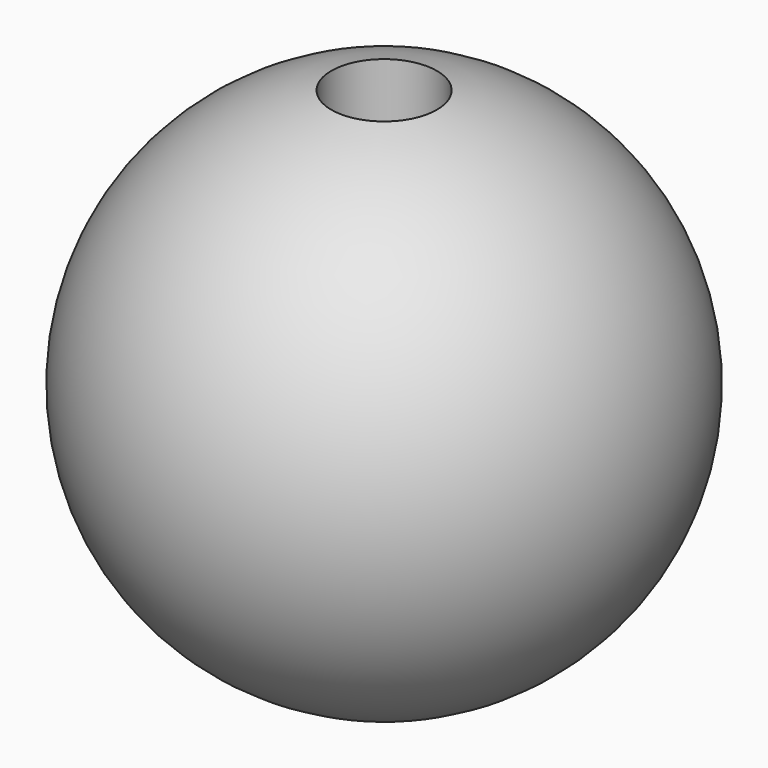
from build123d import *

# Parameters (mm, degrees)
F4_R         = 3.175
F5_DEPTH     = 50.8
F7_ANGLE     = 105.1
F9_TEXT_SIZE = 3.7345061881
F10_DEPTH    = 19.05


# Not quite as in the source:
# - Text() gives the source's letters only with a copy of the font that has no kerning and outlines rounded to 1/6400 em; it was checked with that copy


with BuildPart() as f2:
    # F0 (on Front) → F2 (revolve)
    with BuildSketch(Plane.XZ):
        with BuildLine():
            Line((0, -15.875), (0, 15.875))
            ThreePointArc((0, 15.875), (-15.875, 0), (0, -15.875))
        make_face()
    revolve(axis=Axis((0, 0, 0), (0, 0, 1)))

    # F9 (on offset) → F10 (cut)
    with BuildSketch(Plane(origin=(-24.5230048243, 0, -6.6168145195), x_dir=(0, -1, 0), z_dir=(-0.9654726309, 0, -0.2605045086))):
        with Locations((-4.2756146286, 3.3219258767)):
            Text('105.1', F9_TEXT_SIZE, font='Open Sans', text_align=(TextAlign.LEFT, TextAlign.BOTTOM))
    extrude(amount=-F10_DEPTH, mode=Mode.SUBTRACT)


with BuildPart() as f5:
    # F4 (on offset) → F5 (new body)
    with BuildSketch(Plane.XY.offset(6.35)):
        Circle(F4_R)
    extrude(amount=F5_DEPTH)


with BuildPart() as f7_1:
    # F7: copy of F5
    add(f5.part.rotate(Axis((0, -29.8654846847, 0), (0, -1, 0)), F7_ANGLE))


with BuildPart() as f2_1:
    add(f2.part)

    # F11: cut F5, F7_1
    add(f5.part, mode=Mode.SUBTRACT)
    add(f7_1.part, mode=Mode.SUBTRACT)


solid = f2_1.part
